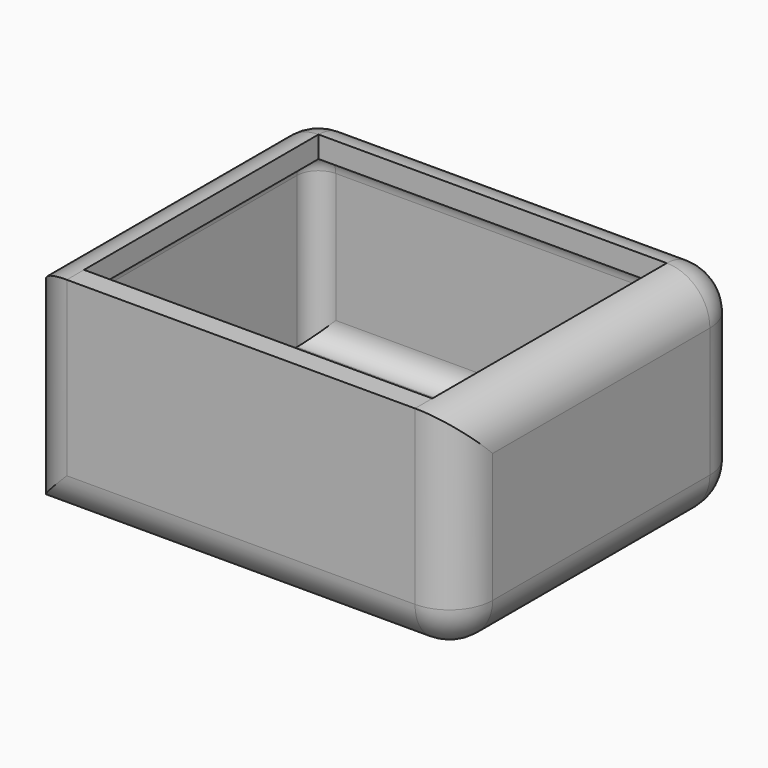
from build123d import *

# Parameters (mm, degrees)
F0_W     = 51.1847995222
F0_H     = 42.1479381621
F1_DEPTH = 25.4
F2_R     = 5.08
F3_T     = -2.54


# Not quite as in the source:
# - a shell that OpenCascade refuses in one call is made with other operations: the cavity is built on its own and cut out


with BuildPart() as f1:
    # F0 (on Top) → F1 (new body)
    with BuildSketch(Plane.XY):
        with Locations((-1.6854219139, -0.4646256566)):
            Rectangle(F0_W, F0_H)
    extrude(amount=F1_DEPTH)

    # F2
    f2_edges = [f1.edges().sort_by_distance(p)[0] for p in [
        (-1.685422, 20.609343, 25.4),
        (-27.277822, -0.464626, 25.4),
        (23.906978, -0.464626, 25.4),
        (23.906978, -0.464626, 0),
        (23.906978, 20.609343, 12.7),
        (23.906978, -21.538595, 12.7),
        (-27.277822, 20.609343, 12.7),
        (-1.685422, -21.538595, 0),
        (-27.277822, -21.538595, 12.7),
        (-1.685422, 20.609343, 0),
    ]]
    fillet(f2_edges, radius=F2_R)

    # F3: a shell. OpenCascade refuses it in one call, so the cavity is built on its own and cut out:
    # the body offset inwards by the wall thickness, plus a prism from it out through each open face.
    f3_core = offset(f1.part, amount=F3_T, mode=Mode.PRIVATE)
    f3_exits = [f3_core.faces().sort_by_distance(p)[0] for p in [
        (-1.685422, -1.734626, 22.86),
    ]]
    add(f3_core, mode=Mode.SUBTRACT)
    extrude(f3_exits, amount=-F3_T, mode=Mode.SUBTRACT)


solid = f1.part
